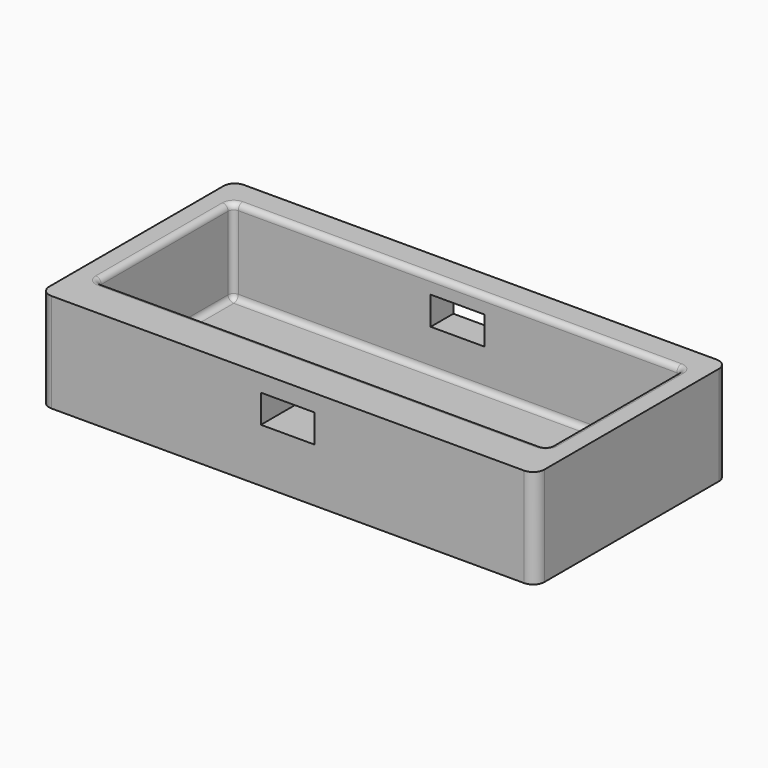
from build123d import *

# Parameters (mm, degrees)
F0_W     = 100.965
F0_H     = 38.1
F1_DEPTH = 19.05
F2_W     = 50.4825
F2_H     = 20.6375
F2_H_2   = 17.4625
F3_DEPTH = 3.175
F4_W     = 12.065
F4_H     = 6.35
F5_DEPTH = 53.976
F6_R     = 1.27


with BuildPart() as f1:
    # F0 (on Top) → F1 (new body)
    with BuildSketch(Plane.XY):
        with BuildLine():
            ThreePointArc((0, 2.54), (0.7439487758, 0.7439487758), (2.54, 0))
            Line((2.54, 0), (108.585, 0))
            ThreePointArc((108.585, 0), (110.3810512242, 0.7439487758), (111.125, 2.54))
            Line((111.125, 2.54), (111.125, 51.435))
            ThreePointArc((111.125, 51.435), (110.3810512242, 53.2310512242), (108.585, 53.975))
            Line((108.585, 53.975), (2.54, 53.975))
            ThreePointArc((2.54, 53.975), (0.7439487758, 53.2310512242), (0, 51.435))
            Line((0, 51.435), (0, 2.54))
        make_face()
        with Locations((55.5625, 28.575)):
            Rectangle(F0_W, F0_H, mode=Mode.SUBTRACT)
    extrude(amount=-F1_DEPTH)

    # F2 (on face) → F3 (join)
    with BuildSketch(Plane(origin=(0, 0, -19.05), x_dir=(1, 0, 0), z_dir=(0, 0, -1))):
        with BuildLine():
            ThreePointArc((0, -51.435), (0.7439487758, -53.2310512242), (2.54, -53.975))
            Line((2.54, -53.975), (55.5625, -53.975))
            Line((55.5625, -53.975), (55.5625, -47.625))
            Line((55.5625, -47.625), (5.08, -47.625))
            Line((5.08, -47.625), (5.08, -26.9875))
            Line((5.08, -26.9875), (0, -26.9875))
            Line((0, -26.9875), (0, -51.435))
        make_face()
        with BuildLine():
            Line((55.5625, -47.625), (55.5625, -53.975))
            Line((55.5625, -53.975), (108.585, -53.975))
            ThreePointArc((108.585, -53.975), (110.3810512242, -53.2310512242), (111.125, -51.435))
            Line((111.125, -51.435), (111.125, -26.9875))
            Line((111.125, -26.9875), (106.045, -26.9875))
            Line((106.045, -26.9875), (106.045, -47.625))
            Line((106.045, -47.625), (55.5625, -47.625))
        make_face()
        with BuildLine():
            Line((0, -2.54), (0, -26.9875))
            Line((0, -26.9875), (5.08, -26.9875))
            Line((5.08, -26.9875), (5.08, -9.525))
            Line((5.08, -9.525), (55.5625, -9.525))
            Line((55.5625, -9.525), (55.5625, 0))
            Line((55.5625, 0), (2.54, 0))
            ThreePointArc((2.54, 0), (0.7439487758, -0.7439487758), (0, -2.54))
        make_face()
        with BuildLine():
            Line((106.045, -26.9875), (111.125, -26.9875))
            Line((111.125, -26.9875), (111.125, -2.54))
            ThreePointArc((111.125, -2.54), (110.3810512242, -0.7439487758), (108.585, 0))
            Line((108.585, 0), (55.5625, 0))
            Line((55.5625, 0), (55.5625, -9.525))
            Line((55.5625, -9.525), (106.045, -9.525))
            Line((106.045, -9.525), (106.045, -26.9875))
        make_face()
        with Locations((30.32125, -37.30625)):
            Rectangle(F2_W, F2_H)
        with Locations((30.32125, -18.25625)):
            Rectangle(F2_W, F2_H_2)
        with Locations((80.80375, -18.25625)):
            Rectangle(F2_W, F2_H_2)
        with Locations((80.80375, -37.30625)):
            Rectangle(F2_W, F2_H)
    extrude(amount=F3_DEPTH)

    # F4 (on face) → F5 (cut, through all)
    with BuildSketch(Plane(origin=(0, 53.975, 0), x_dir=(-1, 0, 0), z_dir=(0, 1, 0))):
        with Locations((-55.5625, -6.985)):
            Rectangle(F4_W, F4_H)
    extrude(amount=-F5_DEPTH, mode=Mode.SUBTRACT)

    # F6
    f6_edges = [f1.edges().sort_by_distance(p)[0] for p in [
        (5.08, 47.625, -9.525),
        (106.045, 47.625, -9.525),
        (5.08, 9.525, -9.525),
        (106.045, 9.525, -9.525),
        (55.5625, 9.525, -19.05),
        (106.045, 28.575, -19.05),
        (55.5625, 47.625, -19.05),
        (5.08, 28.575, -19.05),
        (106.045, 28.575, 0),
        (5.08, 28.575, 0),
        (55.5625, 47.625, 0),
        (55.5625, 9.525, 0),
    ]]
    fillet(f6_edges, radius=F6_R)


solid = f1.part
